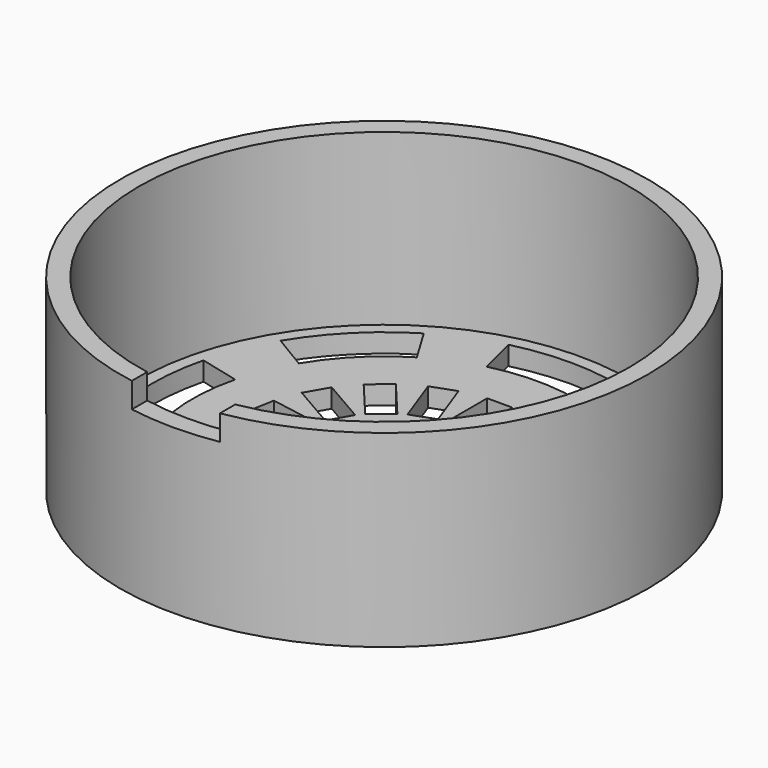
from build123d import *

# Parameters (mm, degrees)
F0_R             = 42
F1_DEPTH         = 3
F2_R             = 42
F2_R_2           = 39
F3_DEPTH         = 27
F5_DEPTH         = 4
F7_DEPTH         = 25.4
F7_COPIES_COUNT  = 8
F8_R             = 10
F9_DEPTH         = 25.4
F10_W            = 4
F10_H            = 8
F11_DEPTH        = 25.4
F11_COPIES_COUNT = 18


# Not quite as in the source:
# - a pattern or mirror of a feature is missing from the dataset's text; its kind, count and spacing are read off the source's solid


with BuildPart() as f1:
    # F0 (on Top) → F1 (new body)
    with BuildSketch(Plane.XY):
        Circle(F0_R)
    extrude(amount=F1_DEPTH)

    # F2 (on face) → F3 (join)
    with BuildSketch(Plane.XY.offset(3)):
        Circle(F2_R)
        Circle(F2_R_2, mode=Mode.SUBTRACT)
    extrude(amount=F3_DEPTH)

    # F4 (on face) → F5 (cut)
    with BuildSketch(Plane.XY.offset(30)):
        with BuildLine():
            ThreePointArc((7, -38.3666521865), (0, -39), (-7, -38.3666521865))
            Line((-7, -38.3666521865), (-7, -41.4125584817))
            ThreePointArc((-7, -41.4125584817), (0, -42), (7, -41.4125584817))
            Line((7, -41.4125584817), (7, -38.3666521865))
        make_face()
    extrude(amount=-F5_DEPTH, mode=Mode.SUBTRACT)

    # F6 (on face) → F7 (cut)
    with BuildSketch(Plane.XY.offset(3)):
        with BuildLine():
            Line((7.3786178158, 29.5940196514), (8.9511101372, 35.9009418722))
            ThreePointArc((8.9511101372, 35.9009418722), (0, 37), (-8.9511101372, 35.9009418722))
            Line((-8.9511101372, 35.9009418722), (-7.3786178158, 29.5940196514))
            ThreePointArc((-7.3786178158, 29.5940196514), (0, 30.5), (7.3786178158, 29.5940196514))
        make_face()
    f7 = extrude(amount=-F7_DEPTH, mode=Mode.SUBTRACT)

    # F7_copies: F7 ×8 about axis
    f7_copies_axis = Axis((0, 0, 0), (0, 0, 1))
    for i in range(1, F7_COPIES_COUNT):
        add(f7.rotate(f7_copies_axis, i * 360 / F7_COPIES_COUNT), mode=Mode.SUBTRACT)

    # F8 (on face) → F9 (cut)
    with BuildSketch(Plane.XY.offset(3)):
        Circle(F8_R)
    extrude(amount=-F9_DEPTH, mode=Mode.SUBTRACT)

    # F10 (on face) → F11 (cut)
    with BuildSketch(Plane.XY.offset(3)):
        with Locations((0, 19)):
            Rectangle(F10_W, F10_H)
    f11 = extrude(amount=-F11_DEPTH, mode=Mode.SUBTRACT)

    # F11_copies: F11 ×18 about axis
    f11_copies_axis = Axis((0, 0, 0), (0, 0, 1))
    for i in range(1, F11_COPIES_COUNT):
        add(f11.rotate(f11_copies_axis, i * 360 / F11_COPIES_COUNT), mode=Mode.SUBTRACT)


solid = f1.part
